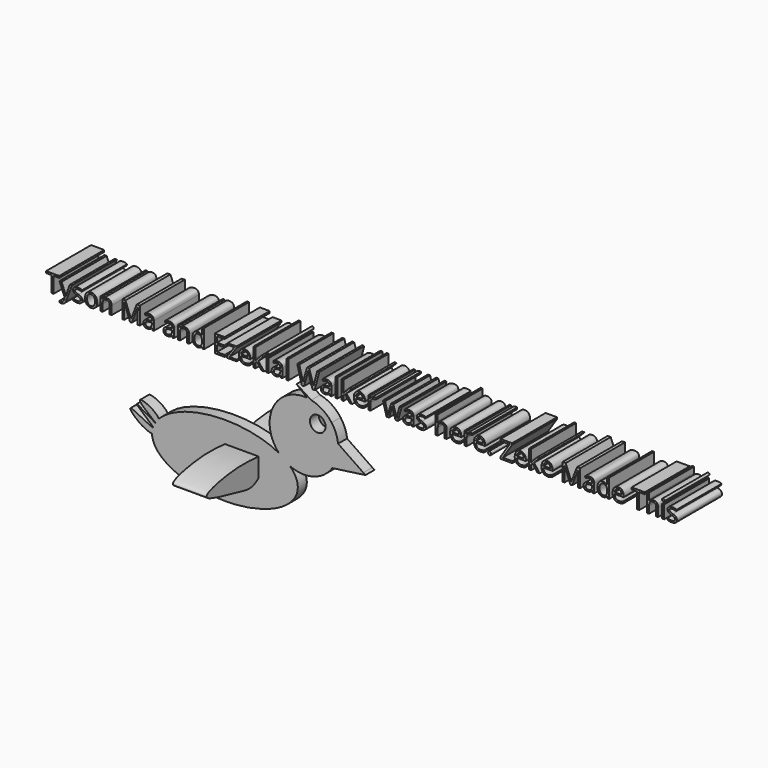
from build123d import *

# Parameters (mm, degrees)
F3_DEPTH     = 15.24
F4_DEPTH     = 5.08
F5_TEXT_SIZE = 11.1050127695
F6_DEPTH     = 25.4


# Not quite as in the source:
# - the program builds the solid bodies; features that only make, move or delete a surface that nothing else refers to are left out
# - Text() gives the source's letters only with a copy of the font that has no kerning and outlines rounded to 1/6400 em; it was checked with that copy


with BuildPart() as f3:
    # F1 (on Right) → F3 (new body)
    with BuildSketch(Plane.YZ):
        with BuildLine():
            add(Edge.make_bspline(
                [(0, -3.0018184334), (5.7922030119, -2.5984744379), (18.7581071903, 1.9356236069), (47.0152799253, -2.8517200481), (23.764169726, -13.7355369078), (13.3248367353, -15.1199163942), (-0.1399536565, -6.2534894348), (-8.0970303043, -15.1180140124), (-16.9422875781, -11.8864792094), (-44.7097207418, -6.9671994335), (-14.0219598499, -0.9536187268), (-5.0956703959, -3.3566589065), (0, -3.0018184334)],
                knots=[0, 0, 0, 0, 0.1194208629, 0.2285173594, 0.3311525609, 0.4217163149, 0.516602977, 0.5936419002, 0.6772288196, 0.7836372533, 0.8949399124, 1, 1, 1, 1], degree=3))
        make_face()
    extrude(amount=F3_DEPTH)

    # F0 (on Front) → F4 (join)
    with BuildSketch(Plane.XZ):
        with BuildLine():
            ThreePointArc((50.7238964132, 8.2425397257), (51.0712900407, 10.1106775656), (51.1876700084, 12.0072737336))
            ThreePointArc((51.1876700084, 12.0072737336), (51.1618612788, 12.9017204052), (51.0845209695, 13.7931907724))
            ThreePointArc((51.0845209695, 13.7931907724), (50.1025065273, 17.7071852117), (48.1441921363, 21.235458101))
            Line((48.1441921363, 21.235458101), (47.3832154511, 18.703635782))
            Line((47.3832154511, 18.703635782), (44.1895796019, 21.4018105136))
            Line((44.1895796019, 21.4018105136), (37.0173549365, 27.4613352294))
            ThreePointArc((37.0173549365, 27.4613352294), (21.7164459878, 18.7729717077), (24.3759328436, 1.379507274))
            add(Edge.make_bspline(
                [(29.3300002621, -2.147720467), (27.333914584, -0.2214232297), (24.3759328436, 1.379507274)],
                knots=[3.6120387141, 3.6120387141, 3.6120387141, 3.878117372, 3.878117372, 3.878117372], degree=2, weights=[1, 0.9911633137, 1]))
            ThreePointArc((29.3300002621, -2.147720467), (39.8793900631, -2.9244261965), (48.473942124, 3.2421426902))
            ThreePointArc((48.473942124, 3.2421426902), (49.8216153086, 5.6421379828), (50.7238964132, 8.2425397257))
        make_face()
        with BuildLine():
            ThreePointArc((45.4422274004, 18.703635782), (38.7062037984, 17.2162493671), (44.1895796019, 21.4018105136))
            ThreePointArc((44.1895796019, 21.4018105136), (45.1137964924, 20.1910221969), (45.4422274004, 18.703635782))
        make_face(mode=Mode.SUBTRACT)
        with BuildLine():
            ThreePointArc((51.0845209695, 13.7931907724), (51.1618612788, 12.9017204052), (51.1876700084, 12.0072737336))
            ThreePointArc((51.1876700084, 12.0072737336), (51.0712900407, 10.1106775656), (50.7238964132, 8.2425397257))
            Line((50.7238964132, 8.2425397257), (62.4843521348, 5.9868156539))
            Line((62.4843521348, 5.9868156539), (51.0845209695, 13.7931907724))
        make_face()
        with BuildLine():
            Line((62.5255977297, 5.2005367167), (50.7238964132, 8.2425397257))
            ThreePointArc((50.7238964132, 8.2425397257), (49.8216153086, 5.6421379828), (48.473942124, 3.2421426902))
            Line((48.473942124, 3.2421426902), (62.5255977297, 5.2005367167))
        make_face()
        Polygon((62.4843521348, 5.9868156539), (50.7238964132, 8.2425397257), (62.5255977297, 5.2005367167), (63.4453743696, 5.3287269548), align=None)
        with BuildLine():
            Line((38.9173401252, 27.1769443532), (48.1441921363, 21.235458101))
            ThreePointArc((48.1441921363, 21.235458101), (44.0737424208, 25.04941817), (38.9173401252, 27.1769443532))
        make_face()
        with BuildLine():
            Line((47.3832154511, 18.703635782), (48.1441921363, 21.235458101))
            Line((48.1441921363, 21.235458101), (38.9173401252, 27.1769443532))
            ThreePointArc((38.9173401252, 27.1769443532), (37.9717544028, 27.3485816341), (37.0173549365, 27.4613352294))
            Line((37.0173549365, 27.4613352294), (44.1895796019, 21.4018105136))
            Line((44.1895796019, 21.4018105136), (47.3832154511, 18.703635782))
        make_face()
        with BuildLine():
            ThreePointArc((37.0173549365, 27.4613352294), (37.9717544028, 27.3485816341), (38.9173401252, 27.1769443532))
            Line((38.9173401252, 27.1769443532), (32.3436111212, 31.4099937677))
            Line((32.3436111212, 31.4099937677), (37.0173549365, 27.4613352294))
        make_face()
        with BuildLine():
            add(Edge.make_bspline(
                [(-32.9045467079, -9.4672730193), (-32.9045467079, -29.9423508925), (7.668729702, -25.1704317036), (48.2420061119, -20.3985125147), (29.3300002621, -2.147720467)],
                knots=[0, 0, 0, 1.8060193571, 1.8060193571, 3.6120387141, 3.6120387141, 3.6120387141], degree=2, weights=[1, 0.6192495943, 1, 0.6192495943, 1]))
            ThreePointArc((29.3300002621, -2.147720467), (26.6784202094, -0.6292606996), (24.3759328436, 1.379507274))
            add(Edge.make_bspline(
                [(24.3759328436, 1.379507274), (-8.8534444598, 19.3640414648), (-29.8070528208, -2.6275665701)],
                knots=[3.878117372, 3.878117372, 3.878117372, 5.8458046955, 5.8458046955, 5.8458046955], degree=2, weights=[1, 0.553826289, 1]))
            add(Edge.make_bspline(
                [(-32.9045467079, -9.4672730193), (-29.5871785013, -9.567963443), (-27.9260766744, -5.6824967661), (-29.8070528208, -2.6275665701)],
                knots=[0.8754804976, 0.8754804976, 0.8754804976, 0.8754804976, 1, 1, 1, 1], degree=3))
        make_face()
        with BuildLine():
            ThreePointArc((24.3759328436, 1.379507274), (26.6784202094, -0.6292606996), (29.3300002621, -2.147720467))
            add(Edge.make_bspline(
                [(29.3300002621, -2.147720467), (27.333914584, -0.2214232297), (24.3759328436, 1.379507274)],
                knots=[3.6120387141, 3.6120387141, 3.6120387141, 3.878117372, 3.878117372, 3.878117372], degree=2, weights=[1, 0.9911633137, 1]))
        make_face()
        with BuildLine():
            add(Edge.make_bspline(
                [(-32.4928506806, -6.9208716131), (-32.72268534, -7.4676631063), (-50.4062087574, 3.2883189421), (-37.084044413, -9.3404148085), (-32.9045467079, -9.4672730193)],
                knots=[0.5685139027, 0.5685139027, 0.5685139027, 0.5685139027, 0.718600422, 0.8754804976, 0.8754804976, 0.8754804976, 0.8754804976], degree=3))
            add(Edge.make_bspline(
                [(-32.4928506806, -6.9208716131), (-32.9045467079, -8.1860571398), (-32.9045467079, -9.4672730193)],
                knots=[6.1248312335, 6.1248312335, 6.1248312335, 6.2831853072, 6.2831853072, 6.2831853072], degree=2, weights=[1, 0.9968671356, 1]))
        make_face()
        with BuildLine():
            add(Edge.make_bspline(
                [(-32.4928506806, -6.9208716131), (-32.9045467079, -8.1860571398), (-32.9045467079, -9.4672730193)],
                knots=[6.1248312335, 6.1248312335, 6.1248312335, 6.2831853072, 6.2831853072, 6.2831853072], degree=2, weights=[1, 0.9968671356, 1]))
            add(Edge.make_bspline(
                [(-32.9045467079, -9.4672730193), (-29.5871785013, -9.567963443), (-27.9260766744, -5.6824967661), (-29.8070528208, -2.6275665701)],
                knots=[0.8754804976, 0.8754804976, 0.8754804976, 0.8754804976, 1, 1, 1, 1], degree=3))
            add(Edge.make_bspline(
                [(-29.8070528208, -2.6275665701), (-30.7742242797, -3.6426497605), (-31.4464247132, -4.7135619811)],
                knots=[5.8458046955, 5.8458046955, 5.8458046955, 5.9843713156, 5.9843713156, 5.9843713156], degree=2, weights=[1, 0.9976008714, 1]))
            add(Edge.make_bspline(
                [(-31.4464247132, -4.7135619811), (-31.4433181339, -4.7240720501), (-31.4468398493, -4.730001777), (-31.4574065674, -4.7310930395)],
                knots=[0.2781978727, 0.2781978727, 0.2781978727, 0.2781978727, 0.2825287093, 0.2825287093, 0.2825287093, 0.2825287093], degree=3))
            add(Edge.make_bspline(
                [(-31.4574065674, -4.7310930395), (-32.1281797541, -5.804061611), (-32.4900409288, -6.9122519104)],
                knots=[5.9855071177, 5.9855071177, 5.9855071177, 6.1242906473, 6.1242906473, 6.1242906473], degree=2, weights=[1, 0.9975933574, 1]))
            add(Edge.make_bspline(
                [(-32.4900409288, -6.9122519104), (-32.490766677, -6.9152706245), (-32.4917039163, -6.9181433868), (-32.4928506806, -6.9208716131)],
                knots=[0.5677650433, 0.5677650433, 0.5677650433, 0.5677650433, 0.5685139027, 0.5685139027, 0.5685139027, 0.5685139027], degree=3))
        make_face()
        with BuildLine():
            add(Edge.make_bspline(
                [(-29.8070528208, -2.6275665701), (-30.7742242797, -3.6426497605), (-31.4464247132, -4.7135619811)],
                knots=[5.8458046955, 5.8458046955, 5.8458046955, 5.9843713156, 5.9843713156, 5.9843713156], degree=2, weights=[1, 0.9976008714, 1]))
            add(Edge.make_bspline(
                [(-29.8070528208, -2.6275665701), (-31.9482338648, 0.8499674958), (-45.1589938624, 5.5629545939), (-31.5443046351, -4.3824180992), (-31.4464247132, -4.7135619811)],
                knots=[0, 0, 0, 0, 0.1417449119, 0.2781978727, 0.2781978727, 0.2781978727, 0.2781978727], degree=3))
        make_face()
        with BuildLine():
            add(Edge.make_bspline(
                [(-32.4900409288, -6.9122519104), (-32.4914481785, -6.9165615754), (-32.4928506806, -6.9208716131)],
                knots=[6.1242906473, 6.1242906473, 6.1242906473, 6.1248312335, 6.1248312335, 6.1248312335], degree=2, weights=[1, 0.9999999635, 1]))
            add(Edge.make_bspline(
                [(-32.4900409288, -6.9122519104), (-32.490766677, -6.9152706245), (-32.4917039163, -6.9181433868), (-32.4928506806, -6.9208716131)],
                knots=[0.5677650433, 0.5677650433, 0.5677650433, 0.5677650433, 0.5685139027, 0.5685139027, 0.5685139027, 0.5685139027], degree=3))
        make_face()
        with BuildLine():
            add(Edge.make_bspline(
                [(-31.4464247132, -4.7135619811), (-31.4433181339, -4.7240720501), (-31.4468398493, -4.730001777), (-31.4574065674, -4.7310930395)],
                knots=[0.2781978727, 0.2781978727, 0.2781978727, 0.2781978727, 0.2825287093, 0.2825287093, 0.2825287093, 0.2825287093], degree=3))
            add(Edge.make_bspline(
                [(-31.4464247132, -4.7135619811), (-31.4519257839, -4.72232598), (-31.4574065674, -4.7310930395)],
                knots=[5.9843713156, 5.9843713156, 5.9843713156, 5.9855071177, 5.9855071177, 5.9855071177], degree=2, weights=[1, 0.9999998387, 1]))
        make_face()
        with BuildLine():
            add(Edge.make_bspline(
                [(-31.4574065674, -4.7310930395), (-31.8012683369, -4.7666048664), (-47.5965511675, 5.5316568956), (-32.3501919761, -6.33055706), (-32.4900409288, -6.9122519104)],
                knots=[0.2825287093, 0.2825287093, 0.2825287093, 0.2825287093, 0.4234626411, 0.5677650433, 0.5677650433, 0.5677650433, 0.5677650433], degree=3))
            add(Edge.make_bspline(
                [(-31.4574065674, -4.7310930395), (-32.1281797541, -5.804061611), (-32.4900409288, -6.9122519104)],
                knots=[5.9855071177, 5.9855071177, 5.9855071177, 6.1242906473, 6.1242906473, 6.1242906473], degree=2, weights=[1, 0.9975933574, 1]))
        make_face()
    extrude(amount=F4_DEPTH)


with BuildPart() as f6:
    # F5 (on Front) → F6 (new body)
    with BuildSketch(Plane.XZ):
        with Locations((-64.5924508572, 45.1542288065)):
            Text('Tyson Ma and Ezekial Walker was here. Zeke Made This', F5_TEXT_SIZE, font='Open Sans', text_align=(TextAlign.LEFT, TextAlign.BOTTOM))
    extrude(amount=F6_DEPTH)


solid = Compound([f3.part, f6.part])
